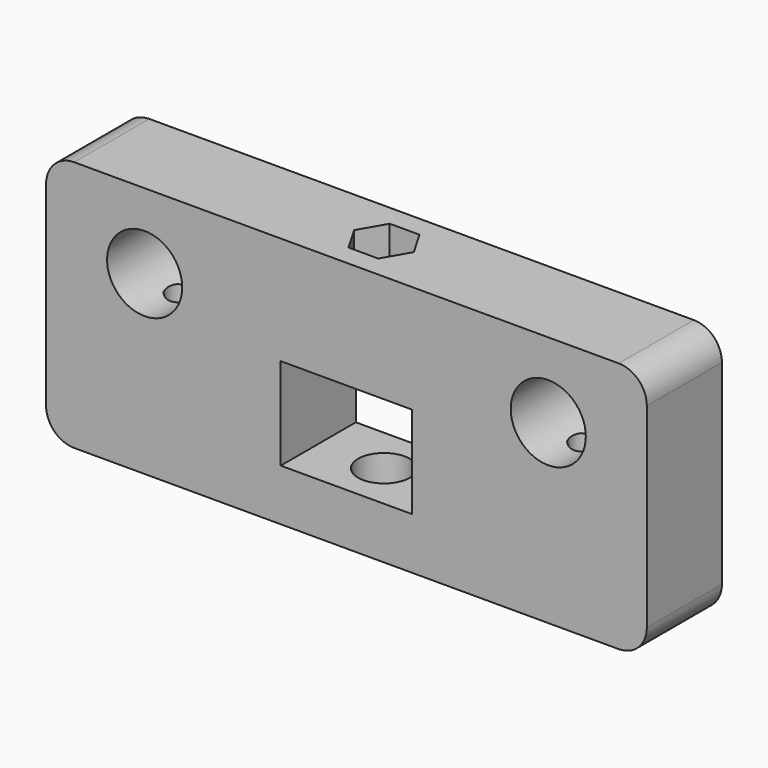
from build123d import *

# Parameters (mm, degrees)
F0_W      = 64
F0_H      = 28
F0_W_2    = 14
F0_H_2    = 9.8
F0_R      = 4
F1_DEPTH  = 5
F1_FACE_W = 64
F1_FACE_H = 10
F4_DEPTH  = 1.2
F5_DEPTH  = 1.2
F7_D      = 3.1
F7_DEPTH  = 15
F7_TIP    = 0.9313339595
F8_R      = 2.75
F9_DEPTH  = 5.5
F10_R     = 1.55
F11_DEPTH = 5
F12_DEPTH = 11.5
F13_R     = 3


# Not quite as in the source:
# - a pattern or mirror of a feature is missing from the dataset's text; its kind, count and spacing are read off the source's solid


with BuildPart() as f1:
    # F0 (on Front) → F1 (new body, symmetric)
    with BuildSketch(Plane.XZ):
        Rectangle(F0_W, F0_H)
        with Locations((0, -2.4)):
            Rectangle(F0_W_2, F0_H_2, mode=Mode.SUBTRACT)
        with Locations((-21.5, 6)):
            Circle(F0_R, mode=Mode.SUBTRACT)
        with Locations((21.5, 6)):
            Circle(F0_R, mode=Mode.SUBTRACT)
    extrude(amount=F1_DEPTH, both=True)

    # F3 (on offset) + F1_face (on face) → F4 (cut, symmetric)
    with BuildSketch(Plane(origin=(0, 0, -4), x_dir=(1, 0, 0), z_dir=(0, 0, -1))):
        Polygon((18.75, 1.5877132403), (18.75, -1.5877132403), (18.75, -5), (24.25, -5), (24.25, 1.5877132403), (21.5, 3.1754264805), align=None)
    with BuildSketch(Plane(origin=(0, 0, -14), x_dir=(1, 0, 0), z_dir=(0, 0, -1))):
        Rectangle(F1_FACE_W, F1_FACE_H)
    extrude(amount=F4_DEPTH, both=True, mode=Mode.SUBTRACT)

    # F3 (on offset) → F5 (cut, symmetric)
    with BuildSketch(Plane(origin=(0, 0, -4), x_dir=(1, 0, 0), z_dir=(0, 0, -1))):
        Polygon((18.75, 1.5877132403), (18.75, -1.5877132403), (18.75, -5), (24.25, -5), (24.25, 1.5877132403), (21.5, 3.1754264805), align=None)
    f5 = extrude(amount=F5_DEPTH, both=True, mode=Mode.SUBTRACT)

    # F5_copies: F5 across plane
    add(f5.mirror(Plane(origin=(0, 0, 0), x_dir=(0, 0, -1), z_dir=(-1, 0, 0))), mode=Mode.SUBTRACT)

    # F7
    with Locations(Plane(origin=(0, 0, -12.8), x_dir=(1, 0, 0), z_dir=(0, 0, -1))):
        with Locations((21.5, 0), (-21.5, 0)):
            Hole(F7_D / 2, depth=F7_DEPTH)
            with Locations((0, 0, -(F7_DEPTH + F7_TIP / 2))):  # 118° drill point
                Cone(0, F7_D / 2, F7_TIP, mode=Mode.SUBTRACT)

    # F8 (on face) → F9 (cut, through all)
    with BuildSketch(Plane(origin=(0, 0, -12.8), x_dir=(1, 0, 0), z_dir=(0, 0, -1))):
        Circle(F8_R)
    extrude(amount=-F9_DEPTH, mode=Mode.SUBTRACT)

    # F10 (on face) → F11 (cut)
    with BuildSketch(Plane.XY.offset(14)):
        Polygon((-1.5877132403, -2.75), (1.5877132403, -2.75), (3.1754264805, 0), (1.5877132403, 2.75), (-1.5877132403, 2.75), (-3.1754264805, 0), align=None)
        Circle(F10_R, mode=Mode.SUBTRACT)
    extrude(amount=-F11_DEPTH, mode=Mode.SUBTRACT)

    # F12 (cut, through all): a face of the model
    f12_faces = [f1.faces().sort_by_distance(p)[0] for p in [
        (0, 0, 14),
    ]]
    extrude(f12_faces, amount=-F12_DEPTH, mode=Mode.SUBTRACT)

    # F13
    f13_edges = [f1.edges().sort_by_distance(p)[0] for p in [
        (32, 0, 14),
        (-32, 0, 14),
        (32, 0, -12.8),
        (-32, 0, -12.8),
    ]]
    fillet(f13_edges, radius=F13_R)


solid = f1.part
